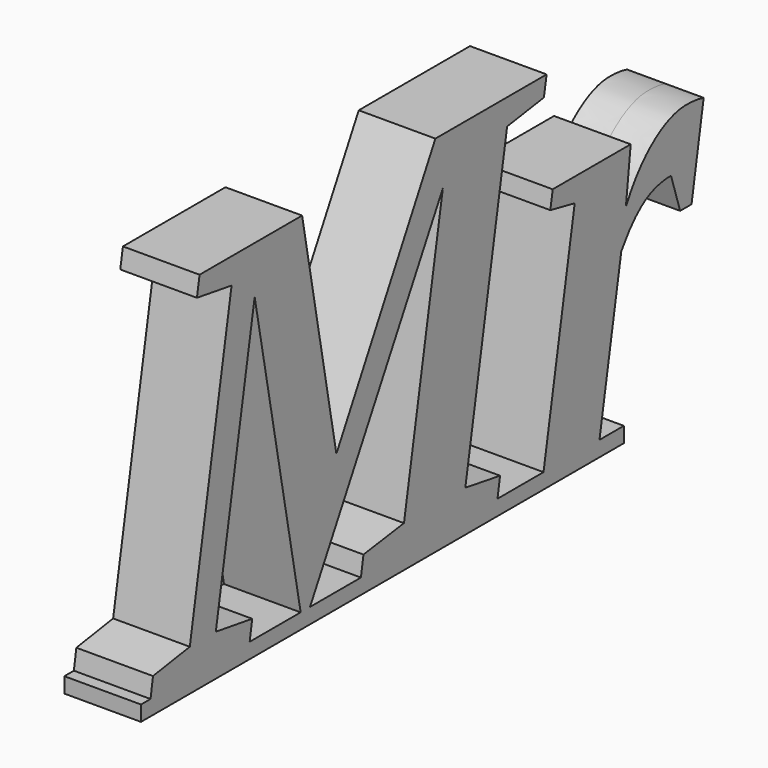
from build123d import *

# Parameters (mm, degrees)
F0_W         = 100
F0_H         = 2.54
F1_DEPTH     = 6.35
F2_TEXT_SIZE = 88.1944444444
F3_DEPTH     = 6.35


# Not quite as in the source:
# - Text() gives the source's letters only with a copy of the font that has no kerning and outlines rounded to 1/6400 em; it was checked with that copy


with BuildPart() as f1:
    # F0 (on Right) → F1 (new body, symmetric)
    with BuildSketch(Plane.YZ):
        with Locations((-30.3918410344, -1.27)):
            Rectangle(F0_W, F0_H)
    extrude(amount=F1_DEPTH, both=True)

    # F2 (on Right) → F3 (join, symmetric)
    with BuildSketch(Plane.YZ):
        with Locations((-77.2574018308, 0)):
            Text('Mr', F2_TEXT_SIZE, font='Tinos', font_style=FontStyle.BOLDITALIC, text_align=(TextAlign.LEFT, TextAlign.BOTTOM))
    extrude(amount=F3_DEPTH, both=True)


solid = f1.part
